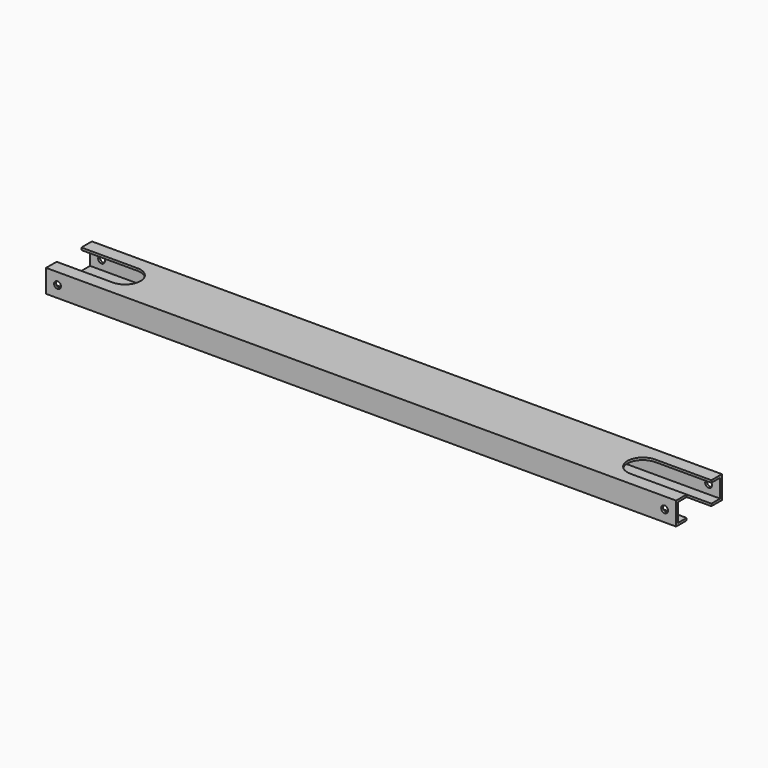
from build123d import *

# Parameters (mm, degrees)
F0_W     = 50
F0_H     = 20
F0_W_2   = 46
F0_H_2   = 16
F1_DEPTH = 550
F2_R     = 3
F3_DEPTH = 50.001
F5_DEPTH = 20.001


# Not quite as in the source:
# - a pattern or mirror of a feature is missing from the dataset's text; its kind, count and spacing are read off the source's solid


with BuildPart() as f1:
    # F0 (on Right) → F1 (new body)
    with BuildSketch(Plane.YZ):
        with Locations((25, 10)):
            Rectangle(F0_W, F0_H)
        with Locations((25, 10)):
            Rectangle(F0_W_2, F0_H_2, mode=Mode.SUBTRACT)
    extrude(amount=F1_DEPTH)

    # F2 (on face) → F3 (cut, through all)
    with BuildSketch(Plane.XZ):
        with Locations((10, 10)):
            Circle(F2_R)
        with Locations((540, 10)):
            Circle(F2_R)
    extrude(amount=-F3_DEPTH, mode=Mode.SUBTRACT)

    # F4 (on face) → F5 (cut, through all)
    with BuildSketch(Plane.XY.offset(20)):
        with BuildLine():
            Line((0, 11.5), (49, 11.5))
            ThreePointArc((49, 11.5), (62.5, 25), (49, 38.5))
            Line((49, 38.5), (0, 38.5))
            Line((0, 38.5), (0, 11.5))
        make_face()
    f5 = extrude(amount=-F5_DEPTH, mode=Mode.SUBTRACT)

    # F5_copies: F5 across plane
    add(f5.mirror(Plane(origin=(275, 0, 0), x_dir=(0, 0, 1), z_dir=(1, 0, 0))), mode=Mode.SUBTRACT)


solid = f1.part
